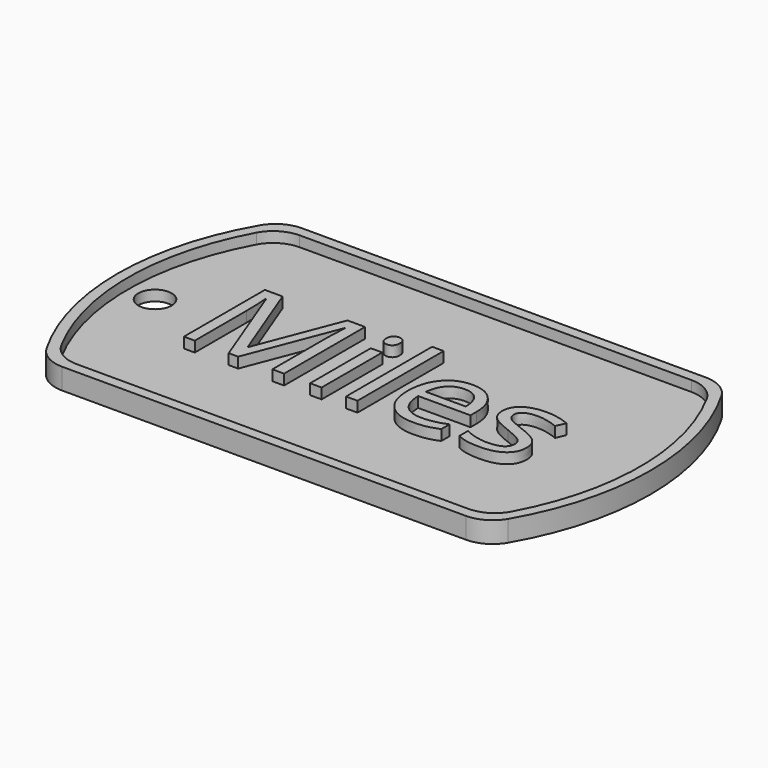
from build123d import *

# Parameters (mm, degrees)
F1_DEPTH     = 1
F3_DEPTH     = 1
F4_R         = 1.5875
F5_DEPTH     = 1
F6_TEXT_SIZE = 13.5061512184
F7_DEPTH     = 1


# Not quite as in the source:
# - the program builds the solid bodies; features that only make, move or delete a surface that nothing else refers to are left out
# - Text() gives the source's letters only with a copy of the font that has no kerning and outlines rounded to 1/6400 em; it was checked with that copy


with BuildPart() as f1:
    # F0 (on Top) → F1 (new body)
    with BuildSketch(Plane.XY):
        with BuildLine():
            ThreePointArc((-19.2474145991, 14.2875), (-20.8349145991, 13.862130657), (-21.9970452561, 12.7))
            ThreePointArc((-21.9970452561, 12.7), (-25.4, 0), (-21.9970452561, -12.7))
            ThreePointArc((-21.9970452561, -12.7), (-20.8349145991, -13.862130657), (-19.2474145991, -14.2875))
            Line((-19.2474145991, -14.2875), (19.2474145991, -14.2875))
            ThreePointArc((19.2474145991, -14.2875), (20.8349145991, -13.862130657), (21.9970452561, -12.7))
            ThreePointArc((21.9970452561, -12.7), (25.4, 0), (21.9970452561, 12.7))
            ThreePointArc((21.9970452561, 12.7), (20.8349145991, 13.862130657), (19.2474145991, 14.2875))
            Line((19.2474145991, 14.2875), (-19.2474145991, 14.2875))
        make_face()
    extrude(amount=F1_DEPTH)

    # F2 (on face) → F3 (join)
    with BuildSketch(Plane.XY.offset(1)):
        with BuildLine():
            Line((19.2474145991, 14.2875), (-19.2474145991, 14.2875))
            ThreePointArc((-19.2474145991, 14.2875), (-20.8349145991, 13.862130657), (-21.9970452561, 12.7))
            ThreePointArc((-21.9970452561, 12.7), (-25.4, 0), (-21.9970452561, -12.7))
            ThreePointArc((-21.9970452561, -12.7), (-20.8349145991, -13.862130657), (-19.2474145991, -14.2875))
            Line((-19.2474145991, -14.2875), (19.2474145991, -14.2875))
            ThreePointArc((19.2474145991, -14.2875), (20.8349145991, -13.862130657), (21.9970452561, -12.7))
            ThreePointArc((21.9970452561, -12.7), (25.4, 0), (21.9970452561, 12.7))
            ThreePointArc((21.9970452561, 12.7), (20.8349145991, 13.862130657), (19.2474145991, 14.2875))
        make_face()
        with BuildLine():
            ThreePointArc((-21.4526124879, 11.6252061249), (-20.2856017842, 12.8404540819), (-18.6611352482, 13.2875))
            Line((-18.6611352482, 13.2875), (18.6611352482, 13.2875))
            ThreePointArc((18.6611352482, 13.2875), (20.2856017842, 12.8404540819), (21.4526124879, 11.6252061249))
            ThreePointArc((21.4526124879, 11.6252061249), (24.4, 0), (21.4526124879, -11.6252061249))
            ThreePointArc((21.4526124879, -11.6252061249), (20.2856017842, -12.8404540819), (18.6611352482, -13.2875))
            Line((18.6611352482, -13.2875), (-18.6611352482, -13.2875))
            ThreePointArc((-18.6611352482, -13.2875), (-20.2856017842, -12.8404540819), (-21.4526124879, -11.6252061249))
            ThreePointArc((-21.4526124879, -11.6252061249), (-24.4, 0), (-21.4526124879, 11.6252061249))
        make_face(mode=Mode.SUBTRACT)
    extrude(amount=F3_DEPTH)

    # F4 (on face) → F5 (cut)
    with BuildSketch(Plane.XY.offset(1)):
        with Locations((-21.821282804, 0)):
            Circle(F4_R)
    extrude(amount=-F5_DEPTH, mode=Mode.SUBTRACT)

    # F6 (on face) → F7 (join)
    with BuildSketch(Plane.XY.offset(1)):
        with Locations((-16.5217537433, -4.8402482644)):
            Text('Miles', F6_TEXT_SIZE, font='Open Sans', text_align=(TextAlign.LEFT, TextAlign.BOTTOM))
    extrude(amount=F7_DEPTH)


solid = f1.part
